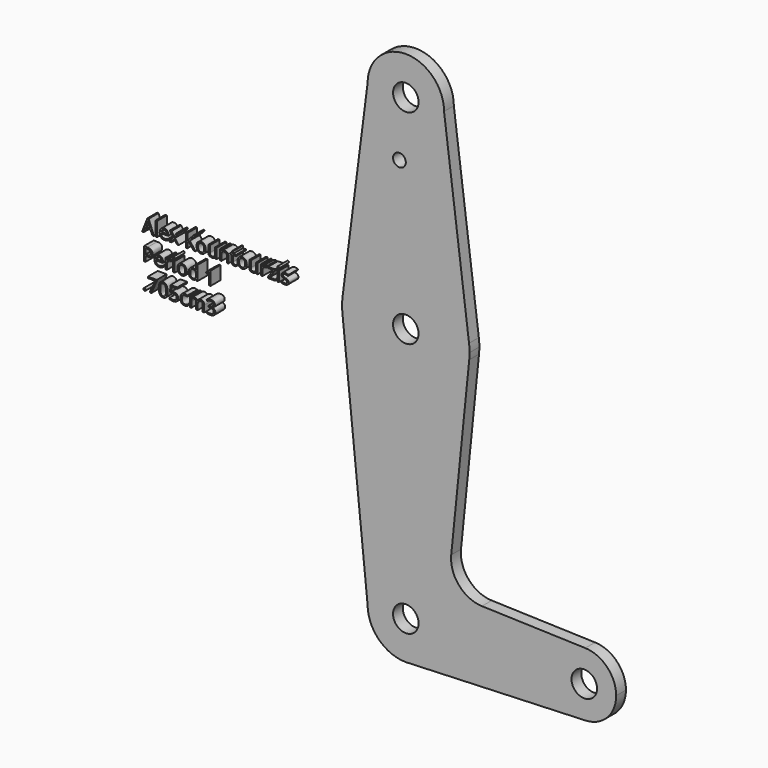
from build123d import *

# Parameters (mm, degrees)
F0_R         = 3.175
F0_R_2       = 1.5875
F0_TEXT_SIZE = 4.6760522916
F1_DEPTH     = 3.048


# Not quite as in the source:
# - Text() gives the source's letters only with a copy of the font that has no kerning and outlines rounded to 1/6400 em; it was checked with that copy


with BuildPart() as f1:
    # F0 (on Front) → F1 (new body)
    with BuildSketch(Plane.XZ):
        with BuildLine():
            ThreePointArc((-9.525, 50.8), (0, 41.275), (9.525, 50.8))
            ThreePointArc((9.525, 50.8), (0, 60.325), (-9.525, 50.8))
        make_face()
        with Locations((0, 50.8)):
            Circle(F0_R, mode=Mode.SUBTRACT)
        with BuildLine():
            Line((15.7474569047, 2.0082893304), (9.525, 50.8))
            ThreePointArc((9.525, 50.8), (0, 41.275), (-9.525, 50.8))
            Line((-9.525, 50.8), (-15.7474569047, 2.0082893304))
            ThreePointArc((-15.7474569047, 2.0082893304), (0, 15.875), (15.7474569047, 2.0082893304))
        make_face()
        with Locations((-1.5875, 36.5252)):
            Circle(F0_R_2, mode=Mode.SUBTRACT)
        with BuildLine():
            ThreePointArc((15.875, 0), (15.8430821396, 1.0061676396), (15.7474569047, 2.0082893304))
            ThreePointArc((15.7474569047, 2.0082893304), (0, 15.875), (-15.7474569047, 2.0082893304))
            ThreePointArc((-15.7474569047, 2.0082893304), (-15.873667691, 0.2056672947), (-15.7942028036, -1.5996195795))
            ThreePointArc((-15.7942028036, -1.5996195795), (-0.0004482141, -15.8749999937), (15.7941124512, -1.6005114426))
            ThreePointArc((15.7941124512, -1.6005114426), (15.8547652169, -0.8012770547), (15.875, 0))
        make_face()
        Circle(F0_R, mode=Mode.SUBTRACT)
        with BuildLine():
            ThreePointArc((15.7941124512, -1.6005114426), (-0.0004482141, -15.8749999937), (-15.7942028036, -1.5996195795))
            Line((-15.7942028036, -1.5996195795), (-9.525, -63.5))
            ThreePointArc((-9.525, -63.5), (0, -53.975), (9.525, -63.5))
            ThreePointArc((9.525, -63.5), (6.9936612334, -69.9663998912), (0.7450887029, -72.9958131734))
            Line((0.7450887029, -72.9958131734), (44.7604045361, -71.2716327043))
            ThreePointArc((44.7604045361, -71.2716327043), (36.5122633209, -63.3685325333), (44.7038065708, -55.4067836673))
            Line((44.7038065708, -55.4067836673), (18.9667787686, -54.582472297))
            ThreePointArc((18.9667787686, -54.582472297), (13.2384784959, -51.8719726214), (11.3115875631, -45.8348107188))
            Line((11.3115875631, -45.8348107188), (15.7941124512, -1.6005114426))
        make_face()
        with BuildLine():
            ThreePointArc((9.525, -63.5), (0, -53.975), (-9.525, -63.5))
            ThreePointArc((-9.525, -63.5), (-6.7351920908, -70.2351920908), (0, -73.025))
            Line((0, -73.025), (0.7450887029, -72.9958131734))
            ThreePointArc((0.7450887029, -72.9958131734), (6.9936612334, -69.9663998912), (9.525, -63.5))
        make_face()
        with Locations((0, -63.5)):
            Circle(F0_R, mode=Mode.SUBTRACT)
        with BuildLine():
            Line((0.7450887029, -72.9958131734), (0, -73.025))
            ThreePointArc((0, -73.025), (0.3728300705, -73.0177004964), (0.7450887029, -72.9958131734))
        make_face()
        with BuildLine():
            ThreePointArc((52.3872128107, -63.340215624), (50.1515009281, -57.8181219527), (44.7038065708, -55.4067836673))
            ThreePointArc((44.7038065708, -55.4067836673), (36.5122633209, -63.3685325333), (44.7604045361, -71.2716327043))
            ThreePointArc((44.7604045361, -71.2716327043), (50.1711646291, -68.841933114), (52.3872128107, -63.340215624))
        make_face()
        with Locations((44.4497128107, -63.340215624)):
            Circle(F0_R, mode=Mode.SUBTRACT)
        with Locations((-65.6894773156, 0)):
            Text('Alex Kountourzis', F0_TEXT_SIZE, font='Open Sans', text_align=(TextAlign.LEFT, TextAlign.BOTTOM))
        with Locations((-65.6894773156, -6.3594311165)):
            Text('Period 1', F0_TEXT_SIZE, font='Open Sans', text_align=(TextAlign.LEFT, TextAlign.BOTTOM))
        with Locations((-65.6894773156, -12.7188622331)):
            Text('.705cm3', F0_TEXT_SIZE, font='Open Sans', text_align=(TextAlign.LEFT, TextAlign.BOTTOM))
    extrude(amount=F1_DEPTH)


solid = f1.part
